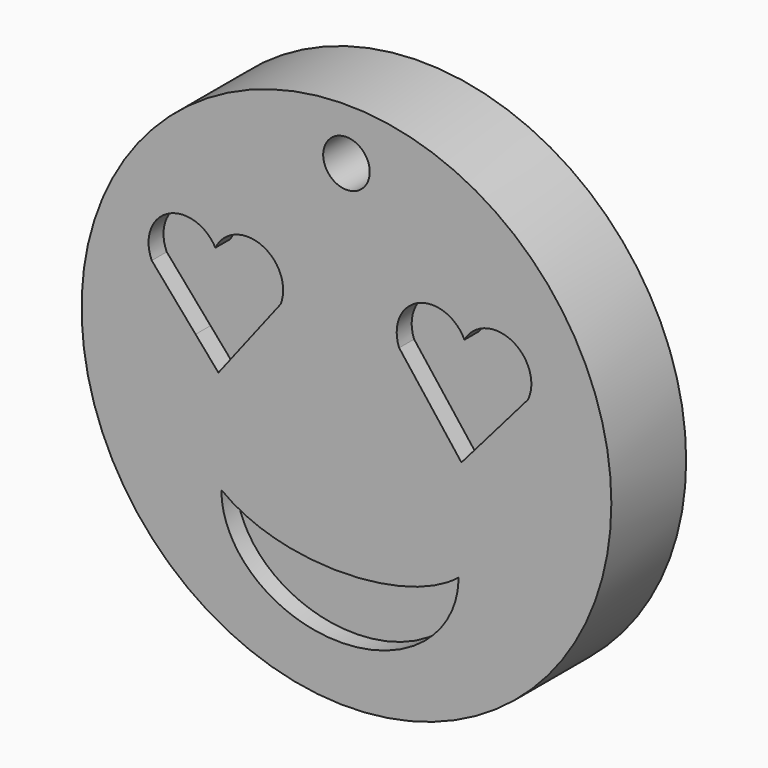
from build123d import *

# Parameters (mm, degrees)
F0_R     = 35.9731805371
F1_DEPTH = 12.7
F3_DEPTH = 2.54
F4_R     = 3.1591269053
F5_DEPTH = 12.7


with BuildPart() as f1:
    # F0 (on Front) → F1 (new body)
    with BuildSketch(Plane.XZ):
        Circle(F0_R)
    extrude(amount=F1_DEPTH)

    # F2 (on face) → F3 (cut)
    with BuildSketch(Plane.XZ.offset(12.7)):
        with BuildLine():
            add(Edge.make_bspline(
                [(-16.9929389652, -15.6046478078), (-8.5501303198, -22.0675654258), (8.323411948, -21.2654638787), (15.2166548375, -15.6046478078)],
                knots=[0, 0, 0, 0, 0.2892568057, 0.2892568057, 0.2892568057, 0.2892568057], degree=3))
            add(Edge.make_bspline(
                [(-16.9929389652, -15.6046478078), (-16.9929389652, -28.5709049037), (-0.8881420638, -28.5709049037), (15.2166548375, -28.5709049037), (15.2166548375, -15.6046478078)],
                knots=[3.1415926536, 3.1415926536, 3.1415926536, 4.7123889804, 4.7123889804, 6.2831853072, 6.2831853072, 6.2831853072], degree=2, weights=[1, 0.7071067812, 1, 0.7071067812, 1]))
        make_face()
        with BuildLine():
            Line((-26.4401481881, 8.735650257), (-20.4888275084, 1.8568773465))
            add(Edge.make_bspline(
                [(-11.8826347663, 5.4031915978), (-15.0818594553, 5.0135593832), (-18.2480697552, 3.9656430572), (-20.2552859644, 2.1019215063), (-20.4888275084, 1.8568773465)],
                knots=[0.7025224358, 0.7025224358, 0.7025224358, 0.7025224358, 0.7815743868, 0.7928961202, 0.7928961202, 0.7928961202, 0.7928961202], degree=3))
            Line((-11.8826347663, 5.4031915978), (-8.9330095374, 9.2211581919))
            ThreePointArc((-8.9330095374, 9.2211581919), (-11.5064602723, 15.4265381827), (-17.8002578016, 13.0776017904))
            ThreePointArc((-17.8002578016, 13.0776017904), (-24.2145633889, 15.0741170918), (-26.4401481881, 8.735650257))
        make_face()
        with BuildLine():
            add(Edge.make_bspline(
                [(-11.8826347663, 5.4031915978), (-15.0818594553, 5.0135593832), (-18.2480697552, 3.9656430572), (-20.2552859644, 2.1019215063), (-20.4888275084, 1.8568773465)],
                knots=[0.7025224358, 0.7025224358, 0.7025224358, 0.7025224358, 0.7815743868, 0.7928961202, 0.7928961202, 0.7928961202, 0.7928961202], degree=3))
            Line((-20.4888275084, 1.8568773465), (-17.3897475746, -1.7251623794))
            Line((-17.3897475746, -1.7251623794), (-11.8826347663, 5.4031915978))
        make_face()
        with BuildLine():
            ThreePointArc((24.6638640604, 8.735650257), (22.4382792612, 15.0741170918), (16.0239736739, 13.0776017904))
            ThreePointArc((16.0239736739, 13.0776017904), (9.7301761446, 15.4265381827), (7.1567254097, 9.2211581919))
            Line((7.1567254097, 9.2211581919), (15.6134634469, -1.7251623794))
            Line((15.6134634469, -1.7251623794), (24.6638640604, 8.735650257))
        make_face()
    extrude(amount=-F3_DEPTH, mode=Mode.SUBTRACT)

    # F4 (on Front) → F5 (cut)
    with BuildSketch(Plane.XZ):
        with Locations((0, 28.9524216205)):
            Circle(F4_R)
    extrude(amount=F5_DEPTH, mode=Mode.SUBTRACT)


solid = f1.part
